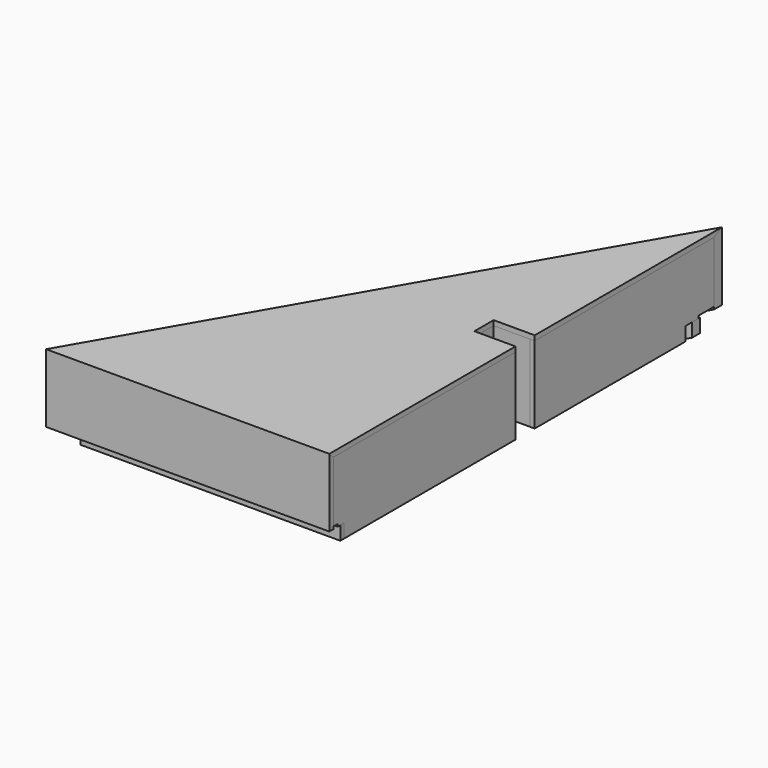
from build123d import *

# Parameters (mm, degrees)
F1_DEPTH      = 250
F2_DEPTH      = 250
F3_DEPTH      = 232
F3_DEPTH_BACK = 50
F0_W          = 18
F0_H          = 88
F4_DEPTH      = 232
F4_DEPTH_BACK = 50
F5_SIZE       = 17.99999
F5_2_SIZE     = 17.99999
F6_W          = 50
F6_H          = 50
F7_DEPTH      = 25
F9_DEPTH      = 50
F11_DEPTH     = 18
F13_DEPTH     = 50
F12_W         = 18
F12_H         = 18
F14_DEPTH     = 50
F17_DEPTH     = 18
F18_SIZE      = 17.99999
F20_DEPTH     = 9


# Not quite as in the source:
# - a fillet or chamfer is up to 0.001 mm smaller than in the source, because OpenCascade refuses the exact size


with BuildPart() as f1:
    # F0 (on Top) → F1 (new body)
    with BuildSketch(Plane.XY):
        Polygon((0, 1793), (-1035, 0), (-1003.8259319586, 18), (-18, 1725.8124599051), (0, 1756.9950686007), align=None)
    extrude(amount=F1_DEPTH)

    # F5 (size 18 in the source; OpenCascade refuses exactly that, so slightly less here)
    f5_edges = [f1.edges().sort_by_distance(p)[0] for p in [
        (-501.912966, 887.497534, 250),
    ]]
    chamfer(f5_edges, length=F5_SIZE)


with BuildPart() as f2:
    # F0 (on Top) → F2 (new body)
    with BuildSketch(Plane.XY):
        Polygon((-1035, 0), (0, 0), (0, 18), (-18, 18), (-1003.8259319586, 18), align=None)
    extrude(amount=F2_DEPTH)

    # F5#2 (size 18 in the source; OpenCascade refuses exactly that, so slightly less here)
    f5_2_edges = [f2.edges().sort_by_distance(p)[0] for p in [
        (-501.912966, 18, 250),
    ]]
    chamfer(f5_2_edges, length=F5_2_SIZE)


with BuildPart() as f3:
    # F0 (on Top) → F3 (new body, two sides)
    with BuildSketch(Plane.XY) as f3_sk:
        Polygon((-18, 18), (0, 18), (0, 850), (-18, 850), (-18, 832), align=None)
    extrude(amount=F3_DEPTH)
    extrude(f3_sk.sketch, amount=-F3_DEPTH_BACK)

    # F6 (on face) → F7 (cut)
    with BuildSketch(Plane.YZ):
        with Locations((43, -25)):
            Rectangle(F6_W, F6_H)
    extrude(amount=-F7_DEPTH, mode=Mode.SUBTRACT)


with BuildPart() as f3b:
    # F0 (on Top) → F3, piece 2 (new body, two sides)
    with BuildSketch(Plane.XY) as f3_2_sk:
        Polygon((0, 938), (0, 1756.9950686007), (-18, 1725.8124599051), (-18, 956), (-18, 938), align=None)
    extrude(amount=F3_DEPTH)
    extrude(f3_2_sk.sketch, amount=-F3_DEPTH_BACK)

    # F8 (on face) → F9 (cut)
    with BuildSketch(Plane(origin=(0, 0, -50), x_dir=(1, 0, 0), z_dir=(0, 0, -1))):
        Polygon((-18, -1625.7987615738), (-18, -1725.8124599051), (0, -1756.9950686007), (0, -1656.9813702694), (0, -1625.7987615738), align=None)
    extrude(amount=-F9_DEPTH, mode=Mode.SUBTRACT)


with BuildPart() as f3c:
    # F0 (on Top) → F3, piece 3 (new body, two sides)
    with BuildSketch(Plane.XY) as f3_3_sk:
        with Locations((-159, 894)):
            Rectangle(F0_W, F0_H)
    extrude(amount=F3_DEPTH)
    extrude(f3_3_sk.sketch, amount=-F3_DEPTH_BACK)


with BuildPart() as f4:
    # F0 (on Top) → F4 (new body, two sides)
    with BuildSketch(Plane.XY) as f4_sk:
        Polygon((-18, 938), (-18, 956), (-168, 956), (-168, 938), (-150, 938), align=None)
    extrude(amount=F4_DEPTH)
    extrude(f4_sk.sketch, amount=-F4_DEPTH_BACK)


with BuildPart() as f4b:
    # F0 (on Top) → F4, piece 2 (new body, two sides)
    with BuildSketch(Plane.XY) as f4_2_sk:
        Polygon((-18, 832), (-18, 850), (-150, 850), (-168, 850), (-168, 832), align=None)
    extrude(amount=F4_DEPTH)
    extrude(f4_2_sk.sketch, amount=-F4_DEPTH_BACK)


with BuildPart() as f11:
    # F10 (on face) → F11 (new body)
    with BuildSketch(Plane(origin=(0, 0, 0), x_dir=(1, 0, 0), z_dir=(0, 0, -1))):
        Polygon((-18, -18), (-1003.8259319586, -18), (-18, -1725.8124599051), (-18, -1625.7987615738), (-18, -956), (-168, -956), (-168, -832), (-18, -832), (-18, -68), align=None)
    extrude(amount=-F11_DEPTH)


with BuildPart() as f13:
    # F12 (on face) → F13 (new body)
    with BuildSketch(Plane(origin=(0, 0, 0), x_dir=(1, 0, 0), z_dir=(0, 0, -1))):
        Polygon((-948.4053665516, -50), (-18, -1661.803692973), (-18, -1625.7987615738), (-917.2312985102, -68), align=None)
        Polygon((-18, -1661.803692973), (0, -1692.9863016687), (0, -1656.9813702694), (-18, -1625.7987615738), align=None)
    extrude(amount=F13_DEPTH)


with BuildPart() as f14:
    # F12 (on face) → F14 (new body)
    with BuildSketch(Plane(origin=(0, 0, 0), x_dir=(1, 0, 0), z_dir=(0, 0, -1))):
        Polygon((-18, -50), (-948.4053665516, -50), (-917.2312985102, -68), (-18, -68), align=None)
        with Locations((-9, -59)):
            Rectangle(F12_W, F12_H)
    extrude(amount=F14_DEPTH)


with BuildPart() as f17:
    # F16 (on offset) → F17 (new body)
    with BuildSketch(Plane.XY.offset(250)):
        Polygon((-1035, 0), (0, 0), (0, 850), (-150, 850), (-150, 938), (0, 938), (0, 1793), align=None)
    extrude(amount=-F17_DEPTH)

    # F18 (size 18 in the source; OpenCascade refuses exactly that, so slightly less here)
    f18_edges = [f17.edges().sort_by_distance(p)[0] for p in [
        (-517.5, 896.5, 232),
        (-517.5, 0, 232),
    ]]
    chamfer(f18_edges, length=F18_SIZE)


with BuildPart() as f20_tool:
    # F19 (on face) → F20 (new body)
    with BuildSketch(Plane(origin=(0, 0, 0), x_dir=(1, 0, 0), z_dir=(0, 0, -1))):
        Polygon((0, -38), (0, -18), (-1003.8259319586, -18), (0, -1756.9950686007), (0, -1685.8069805726), (-18, -1685.8069805726), (-969.1880785792, -38), align=None)
    extrude(amount=-F20_DEPTH)


with BuildPart() as f3_1:
    add(f3.part)

    # F20: cut by f20_tool
    add(f20_tool.part, mode=Mode.SUBTRACT)


with BuildPart() as f3b_1:
    add(f3b.part)

    # F20: cut by f20_tool
    add(f20_tool.part, mode=Mode.SUBTRACT)


with BuildPart() as f11_1:
    add(f11.part)

    # F20: cut by f20_tool
    add(f20_tool.part, mode=Mode.SUBTRACT)


solid = Compound([f1.part, f2.part, f3c.part, f4.part, f4b.part, f13.part, f14.part, f17.part, f3_1.part, f3b_1.part, f11_1.part])
